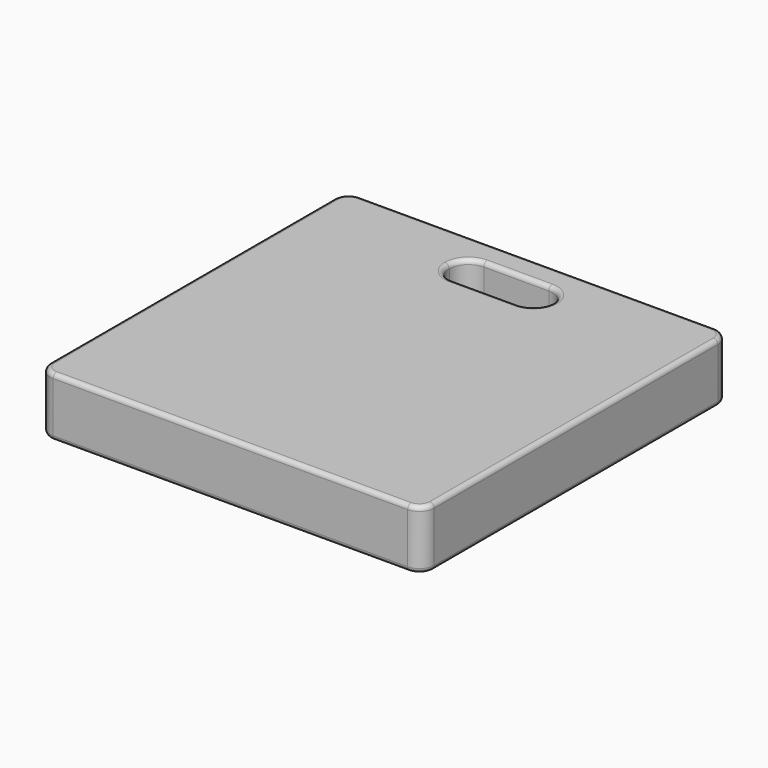
from build123d import *

# Parameters (mm, degrees)
F0_W     = 26
F0_H     = 26
F1_DEPTH = 4
F2_R     = 1
F4_W     = 7
F4_H     = 2.6
F5_DEPTH = 25
F6_R     = 1.29999
F7_R     = 0.3


# Not quite as in the source:
# - a fillet or chamfer is up to 0.001 mm smaller than in the source, because OpenCascade refuses the exact size


with BuildPart() as f1:
    # F0 (on Top) → F1 (new body)
    with BuildSketch(Plane.XY):
        Rectangle(F0_W, F0_H)
    extrude(amount=F1_DEPTH)

    # F2
    f2_edges = [f1.edges().sort_by_distance(p)[0] for p in [
        (-13, -13, 2),
        (-13, 13, 2),
        (13, -13, 2),
        (13, 13, 2),
    ]]
    fillet(f2_edges, radius=F2_R)

    # F4 (on face) → F5 (cut)
    with BuildSketch(Plane.XY.offset(4)):
        with Locations((0, 9.9)):
            Rectangle(F4_W, F4_H)
    extrude(amount=-F5_DEPTH, mode=Mode.SUBTRACT)

    # F6 (radius 1.3 in the source; OpenCascade refuses exactly that, so slightly less here)
    f6_edges = [f1.edges().sort_by_distance(p)[0] for p in [
        (-3.5, 11.2, 2),
        (3.5, 11.2, 2),
        (3.5, 8.6, 2),
        (-3.5, 8.6, 2),
    ]]
    fillet(f6_edges, radius=F6_R)

    # F7
    f7_edges = [f1.edges().sort_by_distance(p)[0] for p in [
        (-13, 0, 4),
        (-13, 0, 0),
        (0, 11.2, 4),
        (0, 11.2, 0),
    ]]
    fillet(f7_edges, radius=F7_R)


solid = f1.part
